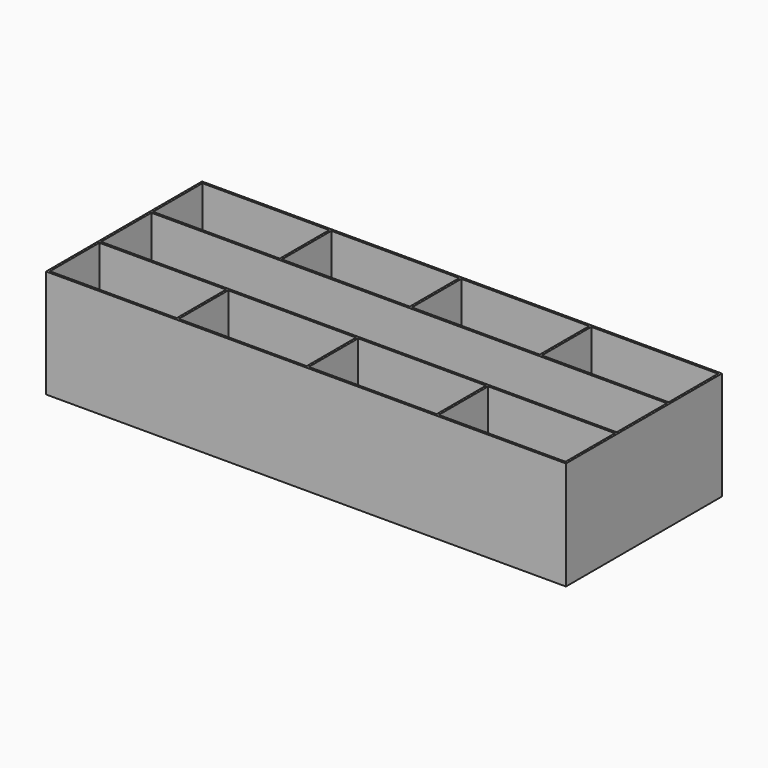
from build123d import *

# Parameters (mm, degrees)
F0_W     = 1200
F0_H     = 450
F1_DEPTH = 250
F2_T     = -5
F3_W     = 5
F3_H     = 142.5
F3_H_2   = 5
F4_DEPTH = 245
F5_R     = 18.5
F6_DEPTH = 25


with BuildPart() as f1:
    # F0 (on Top) → F1 (new body)
    with BuildSketch(Plane.XY):
        Rectangle(F0_W, F0_H)
    extrude(amount=F1_DEPTH)

    # F2
    f2_openings = [f1.faces().sort_by_distance(p)[0] for p in [
        (0, 0, 250),
    ]]
    offset(amount=F2_T, openings=f2_openings)

    # F3 (on face) → F4 (join, through all)
    with BuildSketch(Plane.XY.offset(5)):
        Polygon((302.5, -77.5), (595, -77.5), (595, -72.5), (2.5, -72.5), (-595, -72.5), (-595, -75), (-595, -77.5), (-302.5, -77.5), (-297.5, -77.5), (-2.5, -77.5), (2.5, -77.5), (297.5, -77.5), align=None)
        with Locations((300, -148.75)):
            Rectangle(F3_W, F3_H)
        Polygon((2.5, 72.5), (595, 72.5), (595, 77.5), (302.5, 77.5), (297.5, 77.5), (2.5, 77.5), align=None)
        Polygon((0, -220), (2.5, -220), (2.5, -77.5), (-2.5, -77.5), (-2.5, -220), align=None)
        with Locations((0, 75)):
            Rectangle(F3_W, F3_H_2)
        with Locations((300, 148.75)):
            Rectangle(F3_W, F3_H)
        Polygon((-595, 72.5), (-2.5, 72.5), (-2.5, 77.5), (-297.5, 77.5), (-302.5, 77.5), (-595, 77.5), (-595, 75), align=None)
        with Locations((0, 148.75)):
            Rectangle(F3_W, F3_H)
        Polygon((-297.5, -220), (-297.5, -77.5), (-302.5, -77.5), (-302.5, -220), (-300, -220), align=None)
        with Locations((-300, 148.75)):
            Rectangle(F3_W, F3_H)
    extrude(amount=F4_DEPTH)

    # F5 (on face) → F6 (cut)
    with BuildSketch(Plane.XY.offset(5)):
        with Locations((-42.5, 117.5)):
            Circle(F5_R)
        with Locations((-342.5, 117.5)):
            Circle(F5_R)
        with Locations((-342.5, -117.5)):
            Circle(F5_R)
        with Locations((-42.5, -117.5)):
            Circle(F5_R)
        with Locations((257.5, -117.5)):
            Circle(F5_R)
        with Locations((257.5, 117.5)):
            Circle(F5_R)
        with Locations((555, 117.5)):
            Circle(F5_R)
        with Locations((555, 0)):
            Circle(F5_R)
        with Locations((555, -117.5)):
            Circle(F5_R)
    extrude(amount=-F6_DEPTH, mode=Mode.SUBTRACT)


solid = f1.part
